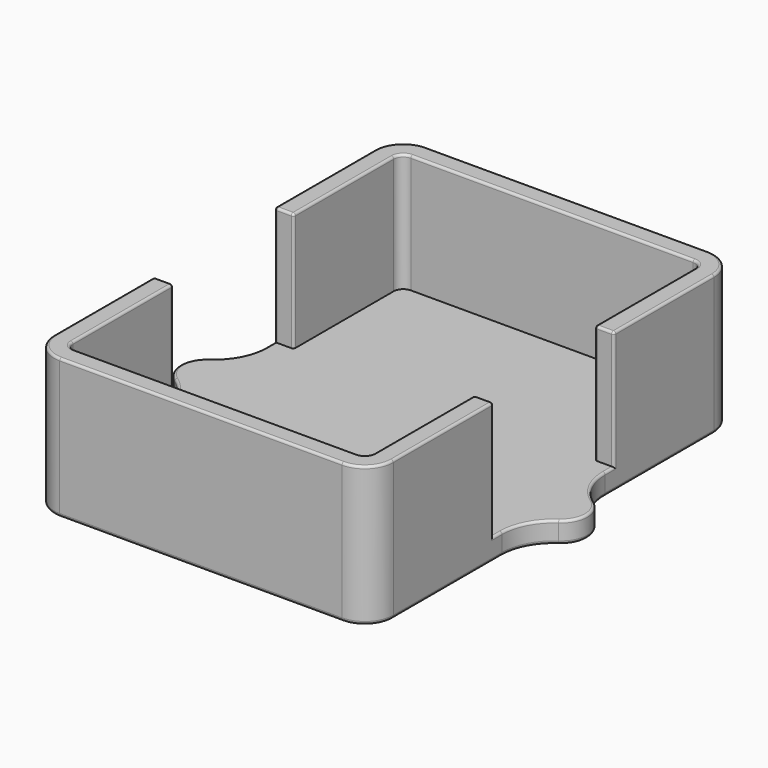
from build123d import *

# Parameters (mm, degrees)
F1_DEPTH  = 4.5
F2_R      = 4.1
F3_DEPTH  = 3.1
F5_DEPTH  = 25
F6_R      = 0.7
F7_R      = 0.5
F8_R      = 0.5
F9_R      = 0.5
F10_R     = 10.1889350931
F11_DEPTH = 25


# Not quite as in the source:
# - ends of sketch curves that miss each other by under 0.0002 mm in the source are joined


with BuildPart() as f1:
    # F0 (on Top) → F1 (new body)
    with BuildSketch(Plane.XY):
        with BuildLine():
            Line((35.75, 13.586758), (35.75, 42.25))
            ThreePointArc((35.75, 42.25), (33.9926406871, 46.4926406871), (29.75, 48.25))
            Line((29.75, 48.25), (-29.75, 48.25))
            ThreePointArc((-29.75, 48.25), (-33.9926406871, 46.4926406871), (-35.75, 42.25))
            Line((-35.75, 42.25), (-35.75, 13.586758))
            ThreePointArc((-35.75, 13.586758), (-37.0008811945, 8.4921841693), (-40.4690331848, 4.5562842657))
            ThreePointArc((-40.4690331848, 4.5562842657), (-42.85, 0), (-40.4690333064, -4.5562844405))
            ThreePointArc((-40.4690333064, -4.5562844405), (-37.0008811945, -8.4921841693), (-35.75, -13.586758))
            Line((-35.75, -13.586758), (-35.75, -42.25))
            ThreePointArc((-35.75, -42.25), (-33.9926406871, -46.4926406871), (-29.75, -48.25))
            Line((-29.75, -48.25), (29.75, -48.25))
            ThreePointArc((29.75, -48.25), (33.9926406871, -46.4926406871), (35.75, -42.25))
            Line((35.75, -42.25), (35.75, -13.586758))
            ThreePointArc((35.75, -13.586758), (37.0008811945, -8.4921841693), (40.4690331848, -4.5562842657))
            ThreePointArc((40.4690331848, -4.5562842657), (42.85, 0), (40.4690333064, 4.5562844405))
            ThreePointArc((40.4690333064, 4.5562844405), (37.0008811945, 8.4921841693), (35.75, 13.586758))
        make_face()
    extrude(amount=F1_DEPTH)

    # F2 (on face) → F3 (cut)
    with BuildSketch(Plane(origin=(0, 0, 0), x_dir=(1, 0, 0), z_dir=(0, 0, -1))):
        with Locations((-37.3, 0)):
            Circle(F2_R)
        with Locations((37.3, 0)):
            Circle(F2_R)
    extrude(amount=-F3_DEPTH, mode=Mode.SUBTRACT)

    # F4 (on face) → F5 (join)
    with BuildSketch(Plane.XY.offset(4.5)):
        with BuildLine():
            Line((-35.75, 42.25), (-35.75, 16.386758))
            ThreePointArc((-35.75, 16.386758), (-35.6035533906, 16.0332046094), (-35.25, 15.886758))
            Line((-35.25, 15.886758), (-32.25, 15.886758))
            ThreePointArc((-32.25, 15.886758), (-31.8964466094, 16.0332046094), (-31.75, 16.386758))
            Line((-31.75, 16.386758), (-31.75, 42.25))
            ThreePointArc((-31.75, 42.25), (-31.1642135624, 43.6642135624), (-29.75, 44.25))
            Line((-29.75, 44.25), (29.75, 44.25))
            ThreePointArc((29.75, 44.25), (31.1642135624, 43.6642135624), (31.75, 42.25))
            Line((31.75, 42.25), (31.75, 16.386758))
            ThreePointArc((31.75, 16.386758), (31.8964466094, 16.0332046094), (32.25, 15.886758))
            Line((32.25, 15.886758), (35.25, 15.886758))
            ThreePointArc((35.25, 15.886758), (35.6035533906, 16.0332046094), (35.75, 16.386758))
            Line((35.75, 16.386758), (35.75, 42.25))
            ThreePointArc((35.75, 42.25), (33.9926406871, 46.4926406871), (29.75, 48.25))
            Line((29.75, 48.25), (-29.75, 48.25))
            ThreePointArc((-29.75, 48.25), (-33.9926406871, 46.4926406871), (-35.75, 42.25))
        make_face()
        with BuildLine():
            Line((35.75, -42.25), (35.75, -16.386758))
            ThreePointArc((35.75, -16.386758), (35.6035533906, -16.0332046094), (35.25, -15.886758))
            Line((35.25, -15.886758), (32.25, -15.886758))
            ThreePointArc((32.25, -15.886758), (31.8964466094, -16.0332046094), (31.75, -16.386758))
            Line((31.75, -16.386758), (31.75, -42.25))
            ThreePointArc((31.75, -42.25), (31.1642135624, -43.6642135624), (29.75, -44.25))
            Line((29.75, -44.25), (-29.75, -44.25))
            ThreePointArc((-29.75, -44.25), (-31.1642135624, -43.6642135624), (-31.75, -42.25))
            Line((-31.75, -42.25), (-31.75, -16.386758))
            ThreePointArc((-31.75, -16.386758), (-31.8964466094, -16.0332046094), (-32.25, -15.886758))
            Line((-32.25, -15.886758), (-35.25, -15.886758))
            ThreePointArc((-35.25, -15.886758), (-35.6035533906, -16.0332046094), (-35.75, -16.386758))
            Line((-35.75, -16.386758), (-35.75, -42.25))
            ThreePointArc((-35.75, -42.25), (-33.9926406871, -46.4926406871), (-29.75, -48.25))
            Line((-29.75, -48.25), (29.75, -48.25))
            ThreePointArc((29.75, -48.25), (33.9926406871, -46.4926406871), (35.75, -42.25))
        make_face()
    extrude(amount=F5_DEPTH)

    # F6
    f6_edges = [f1.edges().sort_by_distance(p)[0] for p in [
        (0, 48.25, 0),
        (-33.992641, 46.492641, 0),
        (-35.75, 27.918379, 0),
        (-37.000881, 8.492184, 0),
        (-42.85, 0, 0),
        (-37.000881, -8.492184, 0),
        (-35.75, -27.918379, 0),
        (-33.992641, -46.492641, 0),
        (0, -48.25, 0),
        (33.992641, -46.492641, 0),
        (35.75, -27.918379, 0),
        (37.000881, -8.492184, 0),
        (42.85, 0, 0),
        (37.000881, 8.492184, 0),
        (35.75, 27.918379, 0),
        (33.992641, 46.492641, 0),
    ]]
    fillet(f6_edges, radius=F6_R)

    # F7
    f7_edges = [f1.edges().sort_by_distance(p)[0] for p in [
        (-33.75, -15.886758, 29.5),
        (-31.896447, -16.033205, 29.5),
        (-31.75, -29.318379, 29.5),
        (-35.603553, -16.033205, 29.5),
        (-35.75, -29.318379, 29.5),
        (-33.992641, -46.492641, 29.5),
        (-31.164214, -43.664214, 29.5),
        (0, -44.25, 29.5),
        (0, -48.25, 29.5),
        (33.992641, -46.492641, 29.5),
        (31.164214, -43.664214, 29.5),
        (31.75, -29.318379, 29.5),
        (35.75, -29.318379, 29.5),
        (35.603553, -16.033205, 29.5),
        (33.75, -15.886758, 29.5),
        (31.896447, -16.033205, 29.5),
        (33.75, 15.886758, 29.5),
        (31.896447, 16.033205, 29.5),
        (31.75, 29.318379, 29.5),
        (35.603553, 16.033205, 29.5),
        (35.75, 29.318379, 29.5),
        (33.992641, 46.492641, 29.5),
        (31.164214, 43.664214, 29.5),
        (0, 44.25, 29.5),
        (0, 48.25, 29.5),
        (-31.164214, 43.664214, 29.5),
        (-33.992641, 46.492641, 29.5),
        (-35.75, 29.318379, 29.5),
        (-31.75, 29.318379, 29.5),
        (-31.896447, 16.033205, 29.5),
        (-33.75, 15.886758, 29.5),
        (-35.603553, 16.033205, 29.5),
    ]]
    fillet(f7_edges, radius=F7_R)

    # F8
    f8_edges = [f1.edges().sort_by_distance(p)[0] for p in [
        (37.000881, -8.492184, 4.5),
        (42.85, 0, 4.5),
        (37.000881, 8.492184, 4.5),
        (35.75, -14.986758, 4.5),
        (35.75, 14.986758, 4.5),
    ]]
    fillet(f8_edges, radius=F8_R)

    # F9
    f9_edges = [f1.edges().sort_by_distance(p)[0] for p in [
        (-35.75, -14.986758, 4.5),
        (-37.000881, -8.492184, 4.5),
        (-42.85, 0, 4.5),
        (-35.75, 14.986758, 4.5),
        (-37.000881, 8.492184, 4.5),
    ]]
    fillet(f9_edges, radius=F9_R)

    # F10 (on face) → F11 (cut)
    with BuildSketch(Plane.XY.offset(4.5)):
        Circle(F10_R)
    extrude(amount=F11_DEPTH, mode=Mode.SUBTRACT)


solid = f1.part
